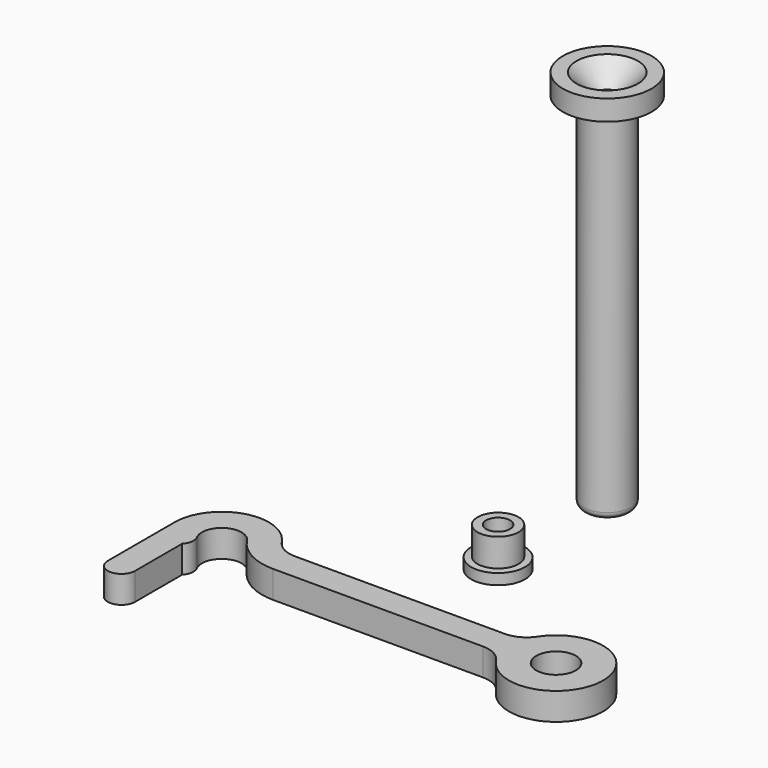
from build123d import *

# Parameters (mm, degrees)
F1_R     = 2.9
F2_DEPTH = 4


# Not quite as in the source:
# - a feature names something its author has since deleted; it is built from what else it names


with BuildPart() as f2:
    # F1 (on Top) → F2 (new body)
    with BuildSketch(Plane.XY):
        with BuildLine():
            Line((15.4, 2), (-15.4, 2))
            ThreePointArc((-15.4, 2), (-17.2963992921, 2.4781156003), (-18.7394495413, 3.7981651376))
            ThreePointArc((-18.7394495413, 3.7981651376), (-26.4827004104, 6.609001368), (-31.4, 0))
            Line((-31.4, 0), (-31.4, -12.2506220506))
            ThreePointArc((-31.4, -12.2506220506), (-29.4, -14.2506220506), (-27.4, -12.2506220506))
            Line((-27.4, -12.2506220506), (-27.4, -3.6254295037))
            ThreePointArc((-27.4, -3.6254295037), (-26.8722153245, -2.5303907614), (-27.0759995835, -1.3320008055))
            ThreePointArc((-27.0759995835, -1.3320008055), (-25.9662125115, 2.5020433392), (-22.0788990826, 1.5963302752))
            ThreePointArc((-22.0788990826, 1.5963302752), (-19.1927985843, -1.0437687994), (-15.4, -2))
            Line((-15.4, -2), (15.4, -2))
            ThreePointArc((15.4, -2), (17.2963992921, -2.4781156003), (18.7394495413, -3.7981651376))
            ThreePointArc((18.7394495413, -3.7981651376), (31.4, 0), (18.7394495413, 3.7981651376))
            ThreePointArc((18.7394495413, 3.7981651376), (17.2963992921, 2.4781156003), (15.4, 2))
        make_face()
        with Locations((24.5, 0)):
            Circle(F1_R, mode=Mode.SUBTRACT)
    extrude(amount=F2_DEPTH)


with BuildPart() as f4:
    # F3 (on Right) → F4 (revolve)
    with BuildSketch(Plane.YZ):
        Polygon((16.05, 1.581099332), (16.05, 0), (16.75, 0), (18.25, 1.5), (18.25, 5.7642135624), (17, 5.7642135624), (17, 1.6642135624), align=None)
    revolve(axis=Axis((0, 20, 5.0162096566), (0, 0, -1)))


with BuildPart() as f5:
    # F3 (on Right) → F5 (revolve)
    with BuildSketch(Plane.YZ):
        with BuildLine():
            Line((36.5, 53), (36.5, 1))
            ThreePointArc((36.5, 1), (37.5, 0), (38.5, 1))
            Line((38.5, 1), (38.5, 53))
            Line((38.5, 53), (35.5, 56))
            Line((35.5, 56), (33.5, 56))
            Line((33.5, 56), (33.5, 53))
            Line((33.5, 53), (36.5, 53))
        make_face()
    revolve(axis=Axis((0, 40, 28.579190366), (0, 0, -1)))


solid = Compound([f2.part, f4.part, f5.part])
